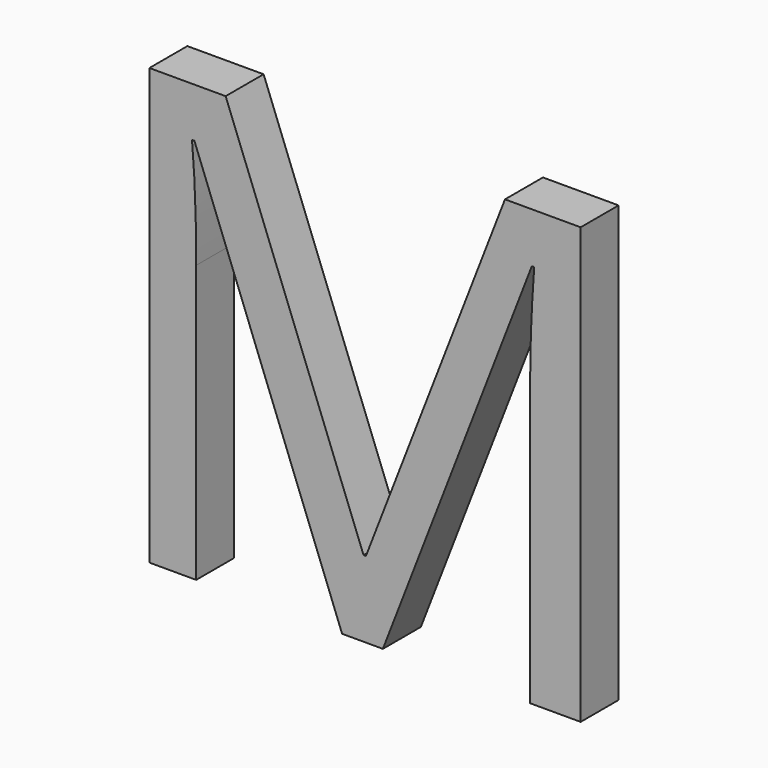
from build123d import *

# Parameters (mm, degrees)
F0_TEXT_SIZE = 97.9562988505
F1_DEPTH     = 7.62


# Not quite as in the source:
# - Text() gives the source's letters only with a copy of the font that has no kerning and outlines rounded to 1/6400 em; it was checked with that copy


with BuildPart() as f1:
    # F0 (on Front) → F1 (new body)
    with BuildSketch(Plane.XZ):
        with Locations((-68.9796432853, -34.3176741153)):
            Text('M', F0_TEXT_SIZE, font='Open Sans', text_align=(TextAlign.LEFT, TextAlign.BOTTOM))
    extrude(amount=F1_DEPTH)


solid = f1.part
